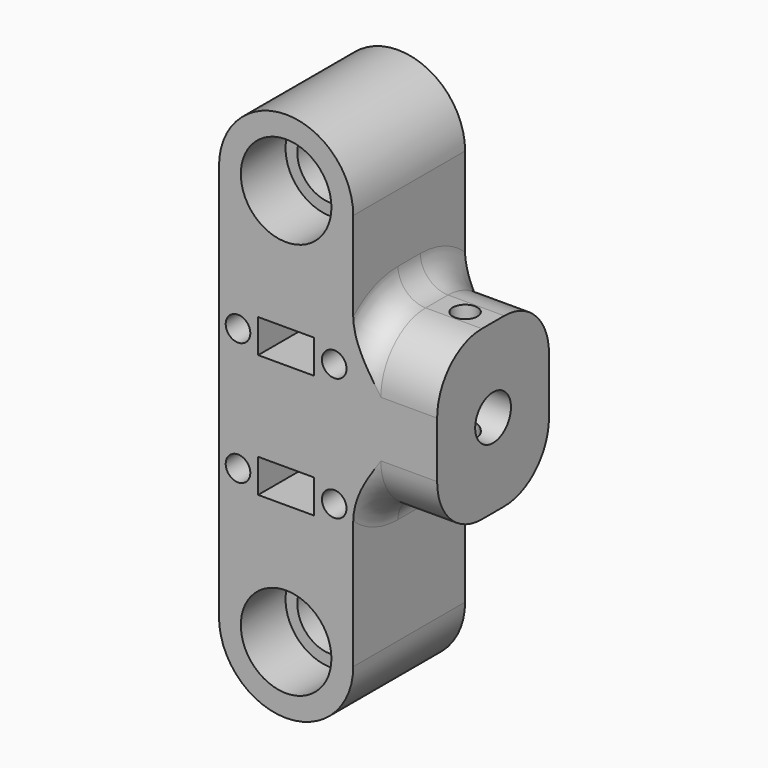
from build123d import *

# Parameters (mm, degrees)
F0_R         = 6
F0_W         = 15
F0_H         = 30
F1_DEPTH     = 25
F2_R         = 8.1
F2_R_2       = 6
F3_DEPTH     = 10
F4_R         = 8.1
F4_R_2       = 6
F5_DEPTH     = 10
F6_R         = 4
F7_DEPTH     = 39.001
F8_R         = 10
F9_T1_DEPTH  = 5
F9_T6_ANGLE  = 161.6623328293
F9_T11_ANGLE = 161.6623328293
F9_T16_ANGLE = 161.6623328293
F9_T21_ANGLE = 161.6623328293
F10_R        = 2.2
F11_DEPTH    = 11.6603414823
F12_R        = 2.2
F13_DEPTH    = 11.6603414823
F14_R        = 1.6
F14_W        = 10
F14_H        = 6
F15_DEPTH    = 25.0010004328
F16_R        = 2.2
F16_R_2      = 1.6
F17_DEPTH    = 6
F18_R        = 2.2
F19_DEPTH    = 6


# Not quite as in the source:
# - a fillet or chamfer that OpenCascade refuses, or shapes differently, is made with other operations: its cross-section is extruded or revolved along the edge and cut away or added


with BuildPart() as f1:
    # F0 (on Front) → F1 (new body)
    with BuildSketch(Plane.XZ):
        with BuildLine():
            Line((12, 18.5), (12, 35.5))
            ThreePointArc((12, 35.5), (0, 23.5), (-12, 35.5))
            Line((-12, 35.5), (-12, -35.5))
            ThreePointArc((-12, -35.5), (0, -23.5), (12, -35.5))
            Line((12, -35.5), (12, -11.5))
            Line((12, -11.5), (12, 18.5))
        make_face()
        with BuildLine():
            ThreePointArc((-12, 35.5), (0, 23.5), (12, 35.5))
            ThreePointArc((12, 35.5), (0, 47.5), (-12, 35.5))
        make_face()
        with Locations((0, 35.5)):
            Circle(F0_R, mode=Mode.SUBTRACT)
        with BuildLine():
            ThreePointArc((12, -35.5), (0, -23.5), (-12, -35.5))
            ThreePointArc((-12, -35.5), (0, -47.5), (12, -35.5))
        make_face()
        with Locations((0, -35.5)):
            Circle(F0_R, mode=Mode.SUBTRACT)
        with Locations((19.5, 3.5)):
            Rectangle(F0_W, F0_H)
    extrude(amount=F1_DEPTH)

    # F2 (on face) → F3 (cut)
    with BuildSketch(Plane.XZ.offset(25)):
        with Locations((0, 35.5)):
            Circle(F2_R)
        with Locations((0, 35.5)):
            Circle(F2_R_2, mode=Mode.SUBTRACT)
        with Locations((0, -35.5)):
            Circle(F2_R)
        with Locations((0, -35.5)):
            Circle(F2_R_2, mode=Mode.SUBTRACT)
    extrude(amount=-F3_DEPTH, mode=Mode.SUBTRACT)

    # F4 (on face) → F5 (cut)
    with BuildSketch(Plane(origin=(0, 0, 0), x_dir=(-1, 0, 0), z_dir=(0, 1, 0))):
        with Locations((0, 35.5)):
            Circle(F4_R)
        with Locations((0, 35.5)):
            Circle(F4_R_2, mode=Mode.SUBTRACT)
        with Locations((0, -35.5)):
            Circle(F4_R)
        with Locations((0, -35.5)):
            Circle(F4_R_2, mode=Mode.SUBTRACT)
    extrude(amount=-F5_DEPTH, mode=Mode.SUBTRACT)

    # F6 (on face) → F7 (cut, through all)
    with BuildSketch(Plane.YZ.offset(27)):
        with Locations((-12.5, 3.5)):
            Circle(F6_R)
    extrude(amount=-F7_DEPTH, mode=Mode.SUBTRACT)

    # F8
    f8_edges = [f1.edges().sort_by_distance(p)[0] for p in [
        (19.5, -25, 18.5),
        (19.5, 0, 18.5),
        (19.5, -25, -11.5),
        (19.5, 0, -11.5),
    ]]
    fillet(f8_edges, radius=F8_R)

    # F9: fillet of radius 5 on 6 edges, made by hand

    # F9_s2 → F9_t1 (join)
    with BuildSketch(Plane.XZ.offset(10)):
        with BuildLine():
            ThreePointArc((11.9996, 23.5009656854), (13.4644660941, 19.9644660941), (17.0009656854, 18.4996))
            Line((17.0009656854, 18.4996), (17.0009656854, 17.9994634315))
            ThreePointArc((17.0009656854, 17.9994634315), (14.5004828427, 17.9998634315), (12, 17.9998634315))
            Line((12, 17.9998634315), (11.4998634315, 18.5))
            ThreePointArc((11.4998634315, 18.5), (11.4998634315, 21.0004828427), (11.4994634315, 23.5009656854))
            Line((11.4994634315, 23.5009656854), (11.9996, 23.5009656854))
        make_face()
        with BuildLine():
            ThreePointArc((11.9996, -16.5009656854), (13.4644660941, -12.9644660941), (17.0009656854, -11.4996))
            Line((17.0009656854, -11.4996), (17.0009656854, -10.9994634315))
            ThreePointArc((17.0009656854, -10.9994634315), (14.5004828427, -10.9998634315), (12, -10.9998634315))
            Line((12, -10.9998634315), (11.4998634315, -11.5))
            ThreePointArc((11.4998634315, -11.5), (11.4998634315, -14.0004828427), (11.4994634315, -16.5009656854))
            Line((11.4994634315, -16.5009656854), (11.9996, -16.5009656854))
        make_face()
    extrude(amount=F9_T1_DEPTH)


with BuildPart() as f9_tool4:
    # F9_s5 → F9_t6 (revolve)
    with BuildSketch(Plane(origin=(0, -6.4717245278, -2.1450392426), x_dir=(1, 0, 0), z_dir=(0, -0.9492188488, -0.3146165557))):
        with BuildLine():
            ThreePointArc((11.9996, -3.7864399137), (13.4644660941, -0.2499403224), (17.0009656854, 1.2149257717))
            Line((17.0009656854, 1.2149257717), (17.0009656854, 1.7150623402))
            ThreePointArc((17.0009656854, 1.7150623402), (14.5004828427, 1.7146623402), (12, 1.7146623402))
            Line((12, 1.7146623402), (11.4998634315, 1.2145257717))
            ThreePointArc((11.4998634315, 1.2145257717), (11.4998634315, -1.285957071), (11.4994634315, -3.7864399137))
            Line((11.4994634315, -3.7864399137), (11.9996, -3.7864399137))
        make_face()
    revolve(axis=Axis((12, -10, 8.5), (1, 0, 0)), revolution_arc=F9_T6_ANGLE)

    split(bisect_by=Plane.XZ, keep=Keep.TOP)


with BuildPart() as f1_1:
    add(f1.part)

    # F9_t3: union F9_tool4
    add(f9_tool4.part)


with BuildPart() as f9_tool9:
    # F9_s10 → F9_t11 (revolve)
    with BuildSketch(Plane(origin=(0, -16.053686044, 5.3209598778), x_dir=(1, 0, 0), z_dir=(0, 0.9492188488, -0.3146165557))):
        with BuildLine():
            ThreePointArc((11.9996, 11.6518538065), (13.4644660941, 8.1153542151), (17.0009656854, 6.650488121))
            Line((17.0009656854, 6.650488121), (17.0009656854, 6.1503515525))
            ThreePointArc((17.0009656854, 6.1503515525), (14.5004828427, 6.1507515525), (12, 6.1507515525))
            Line((12, 6.1507515525), (11.4998634315, 6.650888121))
            ThreePointArc((11.4998634315, 6.650888121), (11.4998634315, 9.1513709638), (11.4994634315, 11.6518538065))
            Line((11.4994634315, 11.6518538065), (11.9996, 11.6518538065))
        make_face()
    revolve(axis=Axis((12, -15, 8.5), (-1, 0, 0)), revolution_arc=F9_T11_ANGLE)

    split(bisect_by=Plane.XZ.offset(25), keep=Keep.BOTTOM)


with BuildPart() as f1_2:
    add(f1_1.part)

    # F9_t8: union F9_tool9
    add(f9_tool9.part)


with BuildPart() as f9_tool14:
    # F9_s15 → F9_t16 (revolve)
    with BuildSketch(Plane(origin=(0, -8.5622042815, 2.8379242825), x_dir=(1, 0, 0), z_dir=(0, -0.9492188488, 0.3146165557))):
        with BuildLine():
            ThreePointArc((17.0009656854, 5.4296061697), (13.4644660941, 6.8944722638), (11.9996, 10.4309718552))
            Line((11.9996, 10.4309718552), (11.4994634315, 10.4309718552))
            ThreePointArc((11.4994634315, 10.4309718552), (11.4998634315, 7.9304890124), (11.4998634315, 5.4300061697))
            Line((11.4998634315, 5.4300061697), (12, 4.9298696012))
            ThreePointArc((12, 4.9298696012), (14.5004828427, 4.9298696012), (17.0009656854, 4.9294696012))
            Line((17.0009656854, 4.9294696012), (17.0009656854, 5.4296061697))
        make_face()
    revolve(axis=Axis((12, -10, -1.5), (-1, 0, 0)), revolution_arc=F9_T16_ANGLE)

    split(bisect_by=Plane.XZ, keep=Keep.TOP)


with BuildPart() as f1_3:
    add(f1_2.part)

    # F9_t13: union F9_tool14
    add(f9_tool14.part)


with BuildPart() as f9_tool19:
    # F9_s20 → F9_t21 (revolve)
    with BuildSketch(Plane(origin=(0, -13.9632062903, -4.6280748379), x_dir=(1, 0, 0), z_dir=(0, 0.9492188488, 0.3146165557))):
        with BuildLine():
            ThreePointArc((11.9996, -18.2963857479), (13.4644660941, -14.7598861565), (17.0009656854, -13.2950200625))
            Line((17.0009656854, -13.2950200625), (17.0009656854, -12.7948834939))
            ThreePointArc((17.0009656854, -12.7948834939), (14.5004828427, -12.7952834939), (12, -12.7952834939))
            Line((12, -12.7952834939), (11.4998634315, -13.2954200625))
            ThreePointArc((11.4998634315, -13.2954200625), (11.4998634315, -15.7959029052), (11.4994634315, -18.2963857479))
            Line((11.4994634315, -18.2963857479), (11.9996, -18.2963857479))
        make_face()
    revolve(axis=Axis((12, -15, -1.5), (1, 0, 0)), revolution_arc=F9_T21_ANGLE)

    split(bisect_by=Plane.XZ.offset(25), keep=Keep.BOTTOM)


with BuildPart() as f1_4:
    add(f1_3.part)

    # F9_t18: union F9_tool19
    add(f9_tool19.part)

    # F10 (on face) → F11 (cut, through all)
    with BuildSketch(Plane.XY.offset(18.5)):
        with Locations((22, -12.5)):
            Circle(F10_R)
    extrude(amount=-F11_DEPTH, mode=Mode.SUBTRACT)

    # F12 (on face) → F13 (cut, through all)
    with BuildSketch(Plane(origin=(0, 0, -11.5), x_dir=(1, 0, 0), z_dir=(0, 0, -1))):
        with Locations((22, 12.5)):
            Circle(F12_R)
    extrude(amount=-F13_DEPTH, mode=Mode.SUBTRACT)

    # F14 (on face) → F15 (cut, through all)
    with BuildSketch(Plane.XZ.offset(25)):
        with Locations((-8.6, 11)):
            Circle(F14_R)
        with Locations((0, 11)):
            Rectangle(F14_W, F14_H)
        with Locations((8.6, 11)):
            Circle(F14_R)
        with Locations((8.6, -11)):
            Circle(F14_R)
        with Locations((0, -11)):
            Rectangle(F14_W, F14_H)
        with Locations((-8.6, -11)):
            Circle(F14_R)
    extrude(amount=-F15_DEPTH, mode=Mode.SUBTRACT)

    # F16 (on face) → F17 (cut)
    with BuildSketch(Plane.XZ.offset(25)):
        with Locations((-8.6, 11)):
            Circle(F16_R)
        with Locations((-8.6, 11)):
            Circle(F16_R_2, mode=Mode.SUBTRACT)
        with Locations((8.6, 11)):
            Circle(F16_R)
        with Locations((8.6, 11)):
            Circle(F16_R_2, mode=Mode.SUBTRACT)
        with Locations((8.6, -11)):
            Circle(F16_R)
        with Locations((8.6, -11)):
            Circle(F16_R_2, mode=Mode.SUBTRACT)
        with Locations((-8.6, -11)):
            Circle(F16_R)
        with Locations((-8.6, -11)):
            Circle(F16_R_2, mode=Mode.SUBTRACT)
    extrude(amount=-F17_DEPTH, mode=Mode.SUBTRACT)

    # F18 (on face) → F19 (cut)
    with BuildSketch(Plane(origin=(0, 0, 0), x_dir=(-1, 0, 0), z_dir=(0, 1, 0))):
        with Locations((8.6, 11)):
            Circle(F18_R)
        with Locations((-8.6, 11)):
            Circle(F18_R)
        with Locations((-8.6, -11)):
            Circle(F18_R)
        with Locations((8.6, -11)):
            Circle(F18_R)
    extrude(amount=-F19_DEPTH, mode=Mode.SUBTRACT)


solid = f1_4.part
